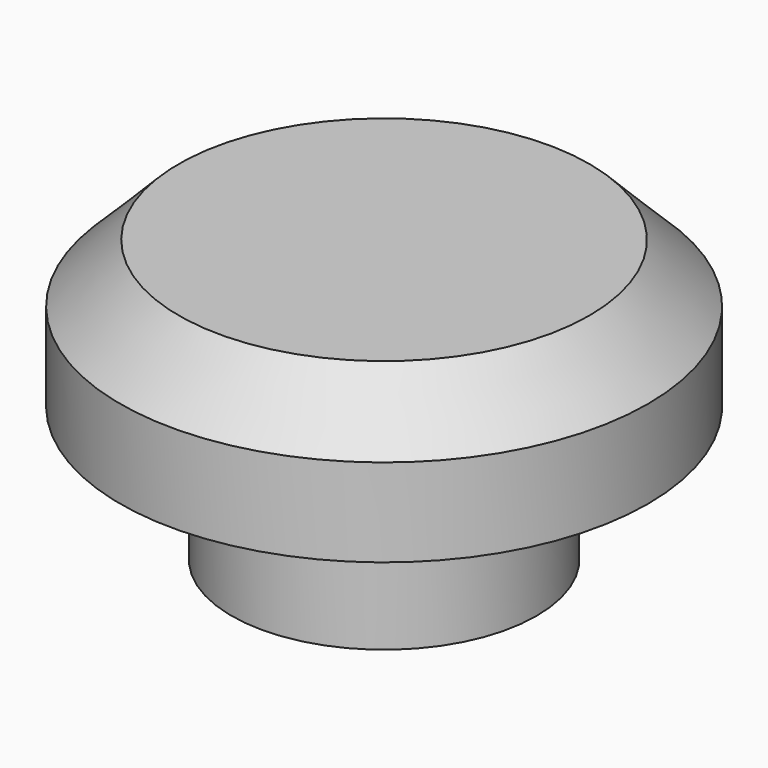
from build123d import *

# Parameters (mm, degrees)
F2_SIZE = 1
F3_SIZE = 0.24999


# Not quite as in the source:
# - a fillet or chamfer is up to 0.001 mm smaller than in the source, because OpenCascade refuses the exact size


with BuildPart() as f1:
    # F0 (on Front) → F1 (revolve)
    with BuildSketch(Plane.XZ):
        Polygon((0, 4.8), (0, 0), (2.6, 0), (2.6, 2.2), (2.35, 2.2), (2.35, 2.3), (2.6, 2.3), (4.5, 2.3), (4.5, 4.8), align=None)
    revolve(axis=Axis((0, 0, 2.4), (0, 0, -1)))

    # F2
    f2_edges = [f1.edges().sort_by_distance(p)[0] for p in [
        (-4.5, 0, 4.8),
    ]]
    chamfer(f2_edges, length=F2_SIZE)

    # F3 (size 0.25 in the source; OpenCascade refuses exactly that, so slightly less here)
    f3_edges = [f1.edges().sort_by_distance(p)[0] for p in [
        (-2.6, 0, 2.2),
    ]]
    chamfer(f3_edges, length=F3_SIZE)


solid = f1.part
